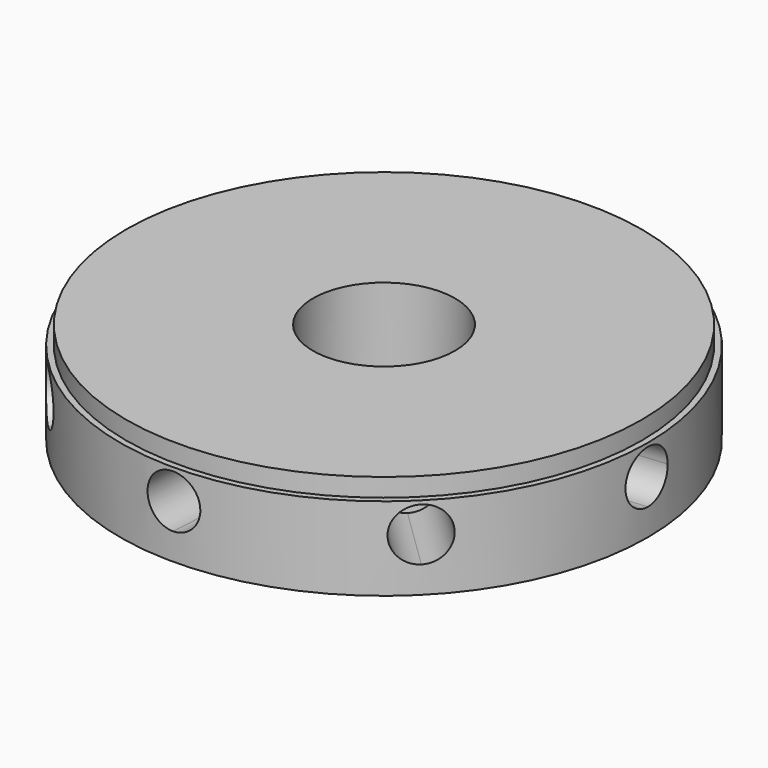
from build123d import *

# Parameters (mm, degrees)
F0_R            = 65
F0_R_2          = 17.5
F1_DEPTH        = 25
F9_DEPTH        = 25
F9_COPIES_COUNT = 8
F10_R           = 65
F10_R_2         = 63.5
F11_DEPTH       = 4.5


# Not quite as in the source:
# - a pattern or mirror of a feature is missing from the dataset's text; its kind, count and spacing are read off the source's solid


with BuildPart() as f1:
    # F0 (on Top) → F1 (new body)
    with BuildSketch(Plane.XY):
        Circle(F0_R)
        Circle(F0_R_2, mode=Mode.SUBTRACT)
    extrude(amount=F1_DEPTH)

    # F8 (on 3pt) → F9 (cut)
    with BuildSketch(Plane(origin=(0, 66.1453359033, 3.4796235199), x_dir=(-1, 0, 0), z_dir=(0, 0.998619184, 0.0525330887))):
        with BuildLine():
            ThreePointArc((0, 3.1838245746), (4.5961940777, 5.0876304969), (6.5, 9.6838245746))
            ThreePointArc((6.5, 9.6838245746), (-4.5961940777, 14.2800186523), (0, 3.1838245746))
        make_face()
    f9 = extrude(amount=-F9_DEPTH, mode=Mode.SUBTRACT)

    # F9_copies: F9 ×8 about axis
    f9_copies_axis = Axis((0, 0, 0), (0, 0, 1))
    for i in range(1, F9_COPIES_COUNT):
        add(f9.rotate(f9_copies_axis, i * 360 / F9_COPIES_COUNT), mode=Mode.SUBTRACT)

    # F10 (on face) → F11 (cut)
    with BuildSketch(Plane.XY.offset(25)):
        Circle(F10_R)
        Circle(F10_R_2, mode=Mode.SUBTRACT)
    extrude(amount=-F11_DEPTH, mode=Mode.SUBTRACT)


solid = f1.part
